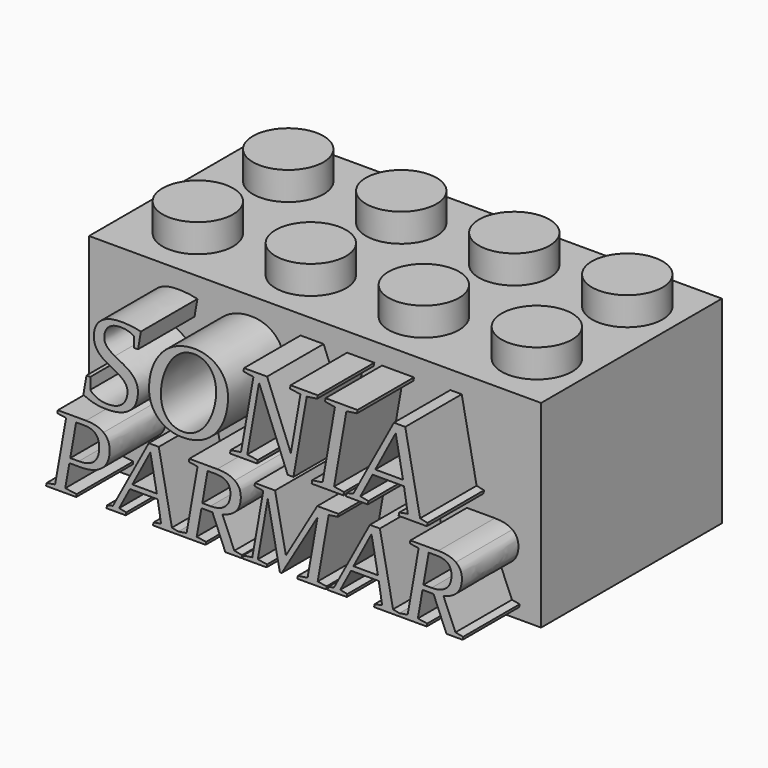
from build123d import *

# Parameters (mm, degrees)
F0_W         = 32
F0_H         = 16
F1_DEPTH     = 14
F2_R         = 2.5
F3_DEPTH     = 2
F4_T         = -2
F5_R         = 3.75
F5_R_2       = 3.25
F6_DEPTH     = 12
F8_DEPTH     = 6.5
F9_TEXT_SIZE = 8.6239422196
F11_DEPTH    = 5
F12_DEPTH    = 5


# Not quite as in the source:
# - Text() gives the source's letters only with a copy of the font that has no kerning and outlines rounded to 1/6400 em; it was checked with that copy


with BuildPart() as f1:
    # F0 (on Top) → F1 (new body)
    with BuildSketch(Plane.XY):
        Rectangle(F0_W, F0_H)
    extrude(amount=F1_DEPTH)

    # F2 (on face) → F3 (join)
    with BuildSketch(Plane.XY.offset(14)):
        with Locations((-11.5, 4)):
            Circle(F2_R)
        with Locations((-3.5, 4)):
            Circle(F2_R)
        with Locations((12.5, 4)):
            Circle(F2_R)
        with Locations((12.5, -4)):
            Circle(F2_R)
        with Locations((4.5, -4)):
            Circle(F2_R)
        with Locations((-3.5, -4)):
            Circle(F2_R)
        with Locations((-11.5, -4)):
            Circle(F2_R)
        with Locations((4.5, 4)):
            Circle(F2_R)
    extrude(amount=F3_DEPTH)

    # F4
    f4_openings = [f1.faces().sort_by_distance(p)[0] for p in [
        (0, 0, 0),
    ]]
    offset(amount=F4_T, openings=f4_openings, kind=Kind.INTERSECTION)

    # F5 (on face) → F6 (join, through all)
    with BuildSketch(Plane(origin=(0, 0, 12), x_dir=(1, 0, 0), z_dir=(0, 0, -1))):
        with Locations((-7.5, 0)):
            Circle(F5_R)
        with Locations((-7.5, 0)):
            Circle(F5_R_2, mode=Mode.SUBTRACT)
        with Locations((0.7, 0)):
            Circle(F5_R)
        with Locations((0.7, 0)):
            Circle(F5_R_2, mode=Mode.SUBTRACT)
        with Locations((8.9, 0)):
            Circle(F5_R)
        with Locations((8.9, 0)):
            Circle(F5_R_2, mode=Mode.SUBTRACT)
    extrude(amount=F6_DEPTH)

    # F7 (on face) → F8 (join)
    with BuildSketch(Plane(origin=(0, 0, 12), x_dir=(1, 0, 0), z_dir=(0, 0, -1))):
        with BuildLine():
            ThreePointArc((-1.3, 3.1721443851), (0.7, 3.75), (2.7, 3.1721443851))
            Line((2.7, 3.1721443851), (2.7, 6))
            Line((2.7, 6), (-1.3, 6))
            Line((-1.3, 6), (-1.3, 3.1721443851))
        make_face()
        with BuildLine():
            Line((2.7, -6), (2.7, -3.1721443851))
            ThreePointArc((2.7, -3.1721443851), (0.7, -3.75), (-1.3, -3.1721443851))
            Line((-1.3, -3.1721443851), (-1.3, -6))
            Line((-1.3, -6), (2.7, -6))
        make_face()
    extrude(amount=F8_DEPTH)

    # F9 (on face) → F11 (join)
    with BuildSketch(Plane.XZ.offset(8)):
        with Locations((-12.5, 7.0221216019)):
            Text('SONIA', F9_TEXT_SIZE, font='Tinos', font_style=FontStyle.ITALIC, text_align=(TextAlign.LEFT, TextAlign.BOTTOM))
    extrude(amount=F11_DEPTH)

    # F10 (on face) → F12 (join)
    with BuildSketch(Plane.XZ.offset(8)):
        with BuildLine():
            Line((-13.6835422949, 1.066211814), (-13.3895413426, 2.7254722488))
            Line((-13.3895413426, 2.7254722488), (-12.6420409459, 2.7254722488))
            add(Edge.make_bspline(
                [(-11.085145215, 3.1640931027), (-11.6302967783, 2.7254722488), (-12.6420409459, 2.7254722488)],
                knots=[0, 0, 0, 1, 1, 1], degree=2))
            add(Edge.make_bspline(
                [(-10.5399936518, 4.4359150357), (-10.5399936518, 3.6027139565), (-11.085145215, 3.1640931027)],
                knots=[0, 0, 0, 1, 1, 1], degree=2))
            add(Edge.make_bspline(
                [(-10.9750436439, 5.4238534582), (-10.5399936518, 5.0905730265), (-10.5399936518, 4.4359150357)],
                knots=[0, 0, 0, 1, 1, 1], degree=2))
            add(Edge.make_bspline(
                [(-12.2135375337, 5.7571338899), (-11.4100936359, 5.7571338899), (-10.9750436439, 5.4238534582)],
                knots=[0, 0, 0, 1, 1, 1], degree=2))
            Line((-12.2135375337, 5.7571338899), (-14.2108395493, 5.7571338899))
            Line((-14.2108395493, 5.7571338899), (-14.2489287415, 5.5595462054))
            Line((-14.2489287415, 5.5595462054), (-13.6240279321, 5.4631329376))
            Line((-13.6240279321, 5.4631329376), (-14.4012855102, 1.066211814))
            Line((-14.4012855102, 1.066211814), (-15.0035708618, 0.9662276845))
            Line((-15.0035708618, 0.9662276845), (-15.0404697667, 0.76864))
            Line((-15.0404697667, 0.76864), (-12.9062847167, 0.76864))
            Line((-12.9062847167, 0.76864), (-12.8681955245, 0.9662276845))
            Line((-12.8681955245, 0.9662276845), (-13.6835422949, 1.066211814))
        make_face()
        with BuildLine():
            add(Edge.make_bspline(
                [(-12.7229804793, 3.0599429678), (-11.280352325, 3.0599429678), (-11.280352325, 4.3883035455)],
                knots=[0, 0, 0, 1, 1, 1], degree=2))
            Line((-12.7229804793, 3.0599429678), (-13.3300269798, 3.0599429678))
            Line((-13.3300269798, 3.0599429678), (-12.9134264402, 5.4214728837))
            Line((-12.9134264402, 5.4214728837), (-12.3623234407, 5.4214728837))
            add(Edge.make_bspline(
                [(-11.5499523885, 5.1709174163), (-11.819552452, 5.4214728837), (-12.3623234407, 5.4214728837)],
                knots=[0, 0, 0, 1, 1, 1], degree=2))
            add(Edge.make_bspline(
                [(-11.280352325, 4.3883035455), (-11.280352325, 4.9203619489), (-11.5499523885, 5.1709174163)],
                knots=[0, 0, 0, 1, 1, 1], degree=2))
        make_face(mode=Mode.SUBTRACT)
        Polygon((-9.4020790351, 0.76864), (-9.3651801301, 0.9662276845), (-9.8674813522, 1.066211814), (-9.1045072211, 2.5052691065), (-7.1405332487, 2.5052691065), (-6.9024757975, 1.066211814), (-7.4345342009, 0.9662276845), (-7.4750039676, 0.76864), (-5.7348039994, 0.76864), (-5.6979050944, 0.9662276845), (-5.6811002576, 0.9690174203), (-6.1323599429, 1.066211814), (-7.0631645771, 5.7976036566), (-7.7725757816, 5.7976036566), (-10.3102682114, 1.066211814), (-10.726868751, 0.9662276845), (-10.7637676559, 0.76864), align=None)
        Polygon((-8.9378670052, 2.8409301127), (-7.658308205, 5.2619743914), (-7.2000476115, 2.8409301127), align=None, mode=Mode.SUBTRACT)
        Polygon((-5.6979050944, 0.9662276845), (-5.7348039994, 0.76864), (-5.7086176797, 0.76864), (-5.668147913, 0.9662276845), (-5.6811002576, 0.9690174203), align=None)
        with BuildLine():
            Line((-5.0956197429, 1.066211814), (-5.6811002576, 0.9690174203))
            Line((-5.6811002576, 0.9690174203), (-5.668147913, 0.9662276845))
            Line((-5.668147913, 0.9662276845), (-5.7086176797, 0.76864))
            Line((-5.7086176797, 0.76864), (-3.7494048564, 0.76864))
            Line((-3.7494048564, 0.76864), (-3.7113156642, 0.9662276845))
            Line((-3.7113156642, 0.9662276845), (-4.3778765275, 1.066211814))
            Line((-4.3778765275, 1.066211814), (-4.0422155213, 2.9563879765))
            Line((-4.0422155213, 2.9563879765), (-3.2649579432, 2.9563879765))
            Line((-3.2649579432, 2.9563879765), (-2.3508173306, 0.76864))
            Line((-2.3508173306, 0.76864), (-1.2045707031, 0.76864))
            Line((-1.2045707031, 0.76864), (-1.1676717981, 0.9662276845))
            Line((-1.1676717981, 0.9662276845), (-1.7140136486, 1.066211814))
            Line((-1.7140136486, 1.066211814), (-2.5591176004, 3.0599429678))
            add(Edge.make_bspline(
                [(-1.2569433423, 4.5478020378), (-1.2569433423, 3.3729885161), (-2.5591176004, 3.0599429678)],
                knots=[0, 0, 0, 1, 1, 1], degree=2))
            add(Edge.make_bspline(
                [(-1.6848516109, 5.4482543469), (-1.2569433423, 5.139374804), (-1.2569433423, 4.5478020378)],
                knots=[0, 0, 0, 1, 1, 1], degree=2))
            add(Edge.make_bspline(
                [(-2.9269163625, 5.7571338899), (-2.1127598794, 5.7571338899), (-1.6848516109, 5.4482543469)],
                knots=[0, 0, 0, 1, 1, 1], degree=2))
            Line((-2.9269163625, 5.7571338899), (-4.9051737819, 5.7571338899))
            Line((-4.9051737819, 5.7571338899), (-4.9432629741, 5.5595462054))
            Line((-4.9432629741, 5.5595462054), (-4.3183621647, 5.4631329376))
            Line((-4.3183621647, 5.4631329376), (-5.0956197429, 1.066211814))
        make_face()
        with BuildLine():
            add(Edge.make_bspline(
                [(-3.4030312649, 3.2908586954), (-2.7257578162, 3.2908586954), (-2.359744485, 3.6122362546)],
                knots=[0, 0, 0, 1, 1, 1], degree=2))
            Line((-3.4030312649, 3.2908586954), (-3.9827011585, 3.2908586954))
            Line((-3.9827011585, 3.2908586954), (-3.6077606729, 5.4214728837))
            Line((-3.6077606729, 5.4214728837), (-3.0566576734, 5.4214728837))
            add(Edge.make_bspline(
                [(-1.9937311538, 4.5251865799), (-1.9937311538, 5.4214728837), (-3.0566576734, 5.4214728837)],
                knots=[0, 0, 0, 1, 1, 1], degree=2))
            add(Edge.make_bspline(
                [(-2.359744485, 3.6122362546), (-1.9937311538, 3.9336138137), (-1.9937311538, 4.5251865799)],
                knots=[0, 0, 0, 1, 1, 1], degree=2))
        make_face(mode=Mode.SUBTRACT)
        Polygon((1.5104745279, 0.76864), (1.6402158388, 0.76864), (4.1731471195, 5.0572449833), (3.4708776385, 1.066211814), (2.7864624663, 0.9662276845), (2.7483732741, 0.76864), (4.7718616093, 0.76864), (4.8099508015, 0.9662276845), (4.1850499921, 1.066211814), (4.9623075702, 5.4631329376), (5.616965561, 5.5595462054), (5.653864466, 5.7571338899), (4.1588636724, 5.7571338899), (1.934216791, 1.9517855325), (1.1676717981, 5.7571338899), (-0.2523408983, 5.7571338899), (-0.2904300905, 5.5595462054), (0.3344707189, 5.4631329376), (-0.4427868592, 1.066211814), (-1.0938739883, 0.9662276845), (-1.1307728932, 0.76864), (0.5653864466, 0.76864), (0.6022853515, 0.9662276845), (-0.0523726393, 1.066211814), (0.651087129, 5.0572449833), align=None)
        Polygon((6.249008094, 0.76864), (6.2859069989, 0.9662276845), (5.7836057769, 1.066211814), (6.546579908, 2.5052691065), (8.5105538803, 2.5052691065), (8.7486113315, 1.066211814), (8.2165529281, 0.9662276845), (8.1760831614, 0.76864), (9.9162831297, 0.76864), (9.9531820346, 0.9662276845), (9.9699868714, 0.9690174203), (9.5187271862, 1.066211814), (8.587922552, 5.7976036566), (7.8785113474, 5.7976036566), (5.3408189176, 1.066211814), (4.924218378, 0.9662276845), (4.8873194731, 0.76864), align=None)
        Polygon((6.7132201238, 2.8409301127), (7.992778924, 5.2619743914), (8.4510395175, 2.8409301127), align=None, mode=Mode.SUBTRACT)
        Polygon((9.9531820346, 0.9662276845), (9.9162831297, 0.76864), (9.9424694493, 0.76864), (9.982939216, 0.9662276845), (9.9699868714, 0.9690174203), align=None)
        with BuildLine():
            Line((10.5554673861, 1.066211814), (9.9699868714, 0.9690174203))
            Line((9.9699868714, 0.9690174203), (9.982939216, 0.9662276845))
            Line((9.982939216, 0.9662276845), (9.9424694493, 0.76864))
            Line((9.9424694493, 0.76864), (11.9016822727, 0.76864))
            Line((11.9016822727, 0.76864), (11.9397714648, 0.9662276845))
            Line((11.9397714648, 0.9662276845), (11.2732106015, 1.066211814))
            Line((11.2732106015, 1.066211814), (11.6088716077, 2.9563879765))
            Line((11.6088716077, 2.9563879765), (12.3861291858, 2.9563879765))
            Line((12.3861291858, 2.9563879765), (13.3002697984, 0.76864))
            Line((13.3002697984, 0.76864), (14.446516426, 0.76864))
            Line((14.446516426, 0.76864), (14.4834153309, 0.9662276845))
            Line((14.4834153309, 0.9662276845), (13.9370734804, 1.066211814))
            Line((13.9370734804, 1.066211814), (13.0919695286, 3.0599429678))
            add(Edge.make_bspline(
                [(14.3941437867, 4.5478020378), (14.3941437867, 3.3729885161), (13.0919695286, 3.0599429678)],
                knots=[0, 0, 0, 1, 1, 1], degree=2))
            add(Edge.make_bspline(
                [(13.9662355182, 5.4482543469), (14.3941437867, 5.139374804), (14.3941437867, 4.5478020378)],
                knots=[0, 0, 0, 1, 1, 1], degree=2))
            add(Edge.make_bspline(
                [(12.7241707665, 5.7571338899), (13.5383272496, 5.7571338899), (13.9662355182, 5.4482543469)],
                knots=[0, 0, 0, 1, 1, 1], degree=2))
            Line((12.7241707665, 5.7571338899), (10.7459133471, 5.7571338899))
            Line((10.7459133471, 5.7571338899), (10.7078241549, 5.5595462054))
            Line((10.7078241549, 5.5595462054), (11.3327249643, 5.4631329376))
            Line((11.3327249643, 5.4631329376), (10.5554673861, 1.066211814))
        make_face()
        with BuildLine():
            add(Edge.make_bspline(
                [(12.2480558641, 3.2908586954), (12.9253293128, 3.2908586954), (13.291342644, 3.6122362546)],
                knots=[0, 0, 0, 1, 1, 1], degree=2))
            Line((12.2480558641, 3.2908586954), (11.6683859705, 3.2908586954))
            Line((11.6683859705, 3.2908586954), (12.0433264561, 5.4214728837))
            Line((12.0433264561, 5.4214728837), (12.5944294556, 5.4214728837))
            add(Edge.make_bspline(
                [(13.6573559752, 4.5251865799), (13.6573559752, 5.4214728837), (12.5944294556, 5.4214728837)],
                knots=[0, 0, 0, 1, 1, 1], degree=2))
            add(Edge.make_bspline(
                [(13.291342644, 3.6122362546), (13.6573559752, 3.9336138137), (13.6573559752, 4.5251865799)],
                knots=[0, 0, 0, 1, 1, 1], degree=2))
        make_face(mode=Mode.SUBTRACT)
    extrude(amount=F12_DEPTH)


solid = f1.part
